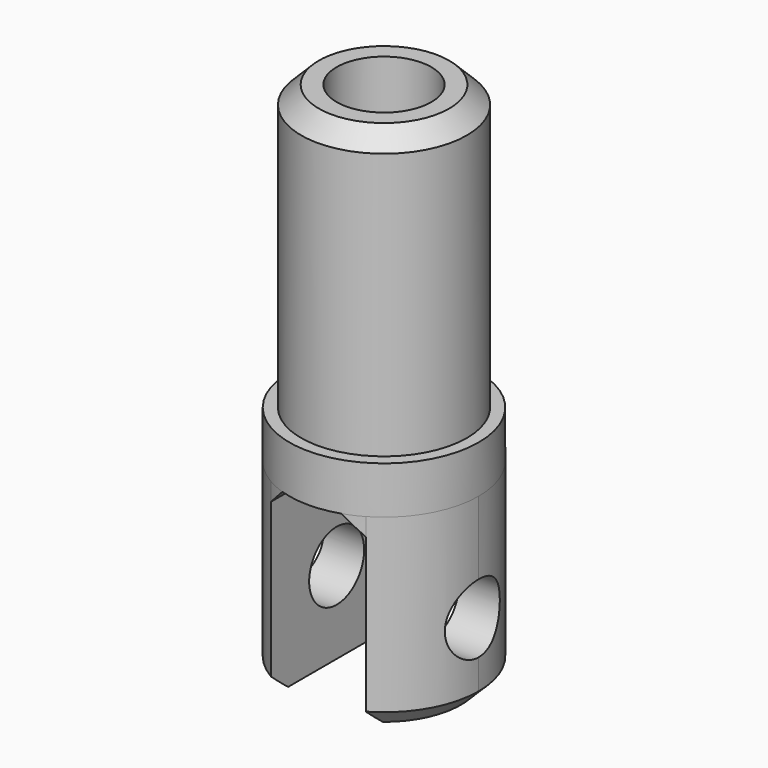
from build123d import *

# Parameters (mm, degrees)
F7_R          = 7
F7_R_2        = 4
F8_DEPTH      = 25
F9_DEPTH      = 1
F7_R_3        = 8
F10_DEPTH     = 1
F11_DEPTH     = 3
F13_DEPTH     = 16
F14_R         = 2.9021632183
F15_DEPTH     = 12.5
F16_T4_DEPTH  = 21.5714554244
F16_S5_R      = 8
F16_T6_DEPTH  = 12
F16_T10_DEPTH = 21.5714554244
F16_S11_R     = 8
F16_T12_DEPTH = 12
F16_T16_ANGLE = 175.2944368931
F16_T18_ANGLE = 175.2944368931


# Not quite as in the source:
# - a fillet or chamfer that OpenCascade refuses, or shapes differently, is made with other operations: its cross-section is extruded or revolved along the edge and cut away or added


with BuildPart() as f8:
    # F7 (on Top) → F8 (new body)
    with BuildSketch(Plane.XY):
        Circle(F7_R)
        Circle(F7_R_2, mode=Mode.SUBTRACT)
    extrude(amount=F8_DEPTH)

    # F7 (on Top) → F9 (join)
    with BuildSketch(Plane.XY):
        Circle(F7_R_2)
    extrude(amount=F9_DEPTH)

    # F7 (on Top) → F10 (join)
    with BuildSketch(Plane.XY):
        Circle(F7_R_3)
        Circle(F7_R, mode=Mode.SUBTRACT)
    extrude(amount=F10_DEPTH)

    # F7 (on Top) → F11 (join)
    with BuildSketch(Plane.XY):
        Circle(F7_R_3)
        Circle(F7_R, mode=Mode.SUBTRACT)
        Circle(F7_R)
        Circle(F7_R_2, mode=Mode.SUBTRACT)
        Circle(F7_R_2)
    extrude(amount=-F11_DEPTH)

    # F12 (on face) → F13 (join)
    with BuildSketch(Plane(origin=(0, 0, -3), x_dir=(1, 0, 0), z_dir=(0, 0, -1))):
        with BuildLine():
            Line((-4, -6.9282032303), (-4, 6.9282032303))
            ThreePointArc((-4, 6.9282032303), (-8, 0), (-4, -6.9282032303))
        make_face()
        with BuildLine():
            ThreePointArc((8, 0), (6.9282032303, 4), (4, 6.9282032303))
            Line((4, 6.9282032303), (4, -6.9282032303))
            ThreePointArc((4, -6.9282032303), (6.9282032303, -4), (8, 0))
        make_face()
    extrude(amount=F13_DEPTH)

    # F14 (on Right) → F15 (cut, symmetric)
    with BuildSketch(Plane.YZ):
        with Locations((0, -12.0717967697)):
            Circle(F14_R)
    extrude(amount=F15_DEPTH, both=True, mode=Mode.SUBTRACT)

    # F16: chamfer of 1.5 on 5 edges, made by hand


with BuildPart() as f16_tool2:
    # F16_s3 → F16_t4 (new body)
    with BuildSketch(Plane.XZ.offset(10.7857277122)):
        Polygon((2.5, -3), (4, -4.5), (4, -3), align=None)
    extrude(amount=-F16_T4_DEPTH)

    # F16_s5 → F16_t6 (intersect, symmetric)
    with BuildSketch(Plane.XY.offset(-3.8)):
        Circle(F16_S5_R)
    extrude(amount=F16_T6_DEPTH, both=True, mode=Mode.INTERSECT)


with BuildPart() as f8_1:
    add(f8.part)

    # F16_t1: union F16_tool2
    add(f16_tool2.part)


with BuildPart() as f16_tool8:
    # F16_s9 → F16_t10 (new body)
    with BuildSketch(Plane.XZ.offset(-10.7857277122)):
        Polygon((-2.5, -3), (-4, -4.5), (-4, -3), align=None)
    extrude(amount=F16_T10_DEPTH)

    # F16_s11 → F16_t12 (intersect, symmetric)
    with BuildSketch(Plane.XY.offset(-3.8)):
        Circle(F16_S11_R)
    extrude(amount=F16_T12_DEPTH, both=True, mode=Mode.INTERSECT)


with BuildPart() as f8_2:
    add(f8_1.part)

    # F16_t7: union F16_tool8
    add(f16_tool8.part)

    # F16_s13 → F16_t14 (revolve, cut)
    with BuildSketch(Plane.XZ):
        Polygon((7, 23.5), (5.5, 25), (7, 25), align=None)
    revolve(axis=Axis((0, 0, 25), (0, 0, 1)), mode=Mode.SUBTRACT)

    # F16_s15 → F16_t16 (revolve, cut)
    with BuildSketch(Plane(origin=(0, 0, 0), x_dir=(0, 0, 1), z_dir=(-0.9991570013, 0.0410522451, 0))):
        Polygon((-17.5, 8), (-19, 6.5), (-19, 8), align=None)
    revolve(axis=Axis((0, 0, -19), (0, 0, -1)), revolution_arc=F16_T16_ANGLE, mode=Mode.SUBTRACT)

    # F16_s17 → F16_t18 (revolve, cut)
    with BuildSketch(Plane(origin=(0, 0, 0), x_dir=(0, 0, 1), z_dir=(0.9991570013, -0.0410522451, 0))):
        Polygon((-17.5, 8), (-19, 6.5), (-19, 8), align=None)
    revolve(axis=Axis((0, 0, -19), (0, 0, -1)), revolution_arc=F16_T18_ANGLE, mode=Mode.SUBTRACT)


solid = f8_2.part
